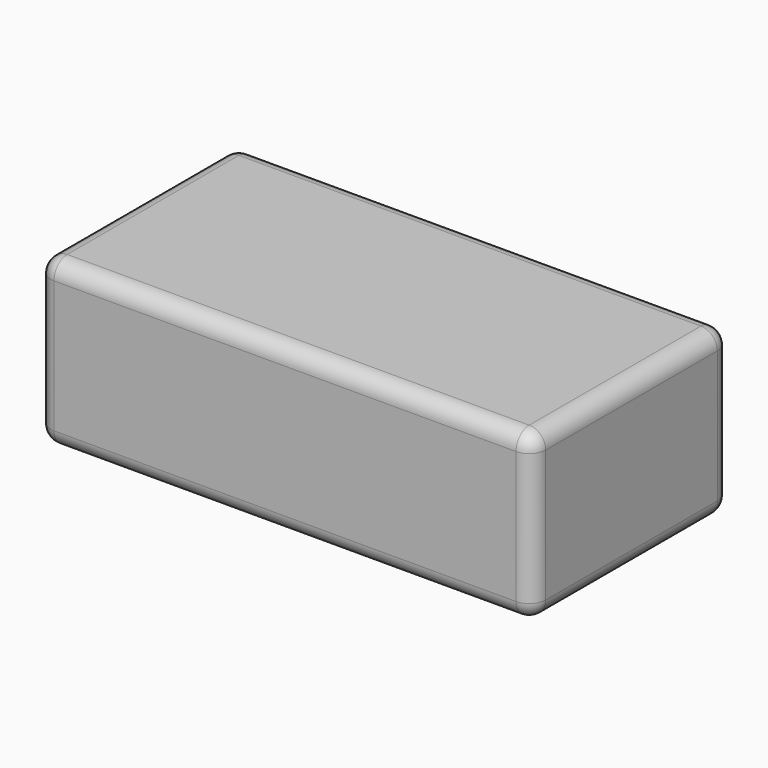
from build123d import *

# Parameters (mm, degrees)
F0_W          = 152.4
F0_H          = 76.2
F1_DEPTH      = 50.8
F2_R          = 18.0745305817
F3_DEPTH      = 38.1
F6_DEPTH      = 38.1
F4_W          = 35.56
F4_H          = 35.56
F7_DEPTH      = 38.1
F8_T1_DEPTH   = 35.56
F8_T3_DEPTH   = 35.56
F8_T5_DEPTH   = 142.24
F8_T7_DEPTH   = 66.04
F8_T9_DEPTH   = 40.64
F8_S13_W      = 5.08
F8_S13_H      = 5.08
F8_T14_DEPTH  = 5.08
F8_S19_W      = 5.08
F8_S19_H      = 5.08
F8_T20_DEPTH  = 5.08
F8_S25_W      = 5.08
F8_S25_H      = 5.08
F8_T26_DEPTH  = 5.08
F8_S31_W      = 5.08
F8_S31_H      = 5.08
F8_T32_DEPTH  = 5.08
F8_S37_W      = 5.08
F8_S37_H      = 5.08
F8_T38_DEPTH  = 5.08
F8_S43_W      = 5.08
F8_S43_H      = 5.08
F8_T44_DEPTH  = 5.08
F8_S49_W      = 5.08
F8_S49_H      = 5.08
F8_T50_DEPTH  = 5.08
F8_S55_W      = 5.08
F8_S55_H      = 5.08
F8_T56_DEPTH  = 5.08
F8_T64_DEPTH  = 64.7384888256
F8_T70_DEPTH  = 64.7384888256
F8_T76_DEPTH  = 55.6341915667
F8_T83_DEPTH  = 48.26
F8_T87_DEPTH  = 48.26
F8_T94_DEPTH  = 48.26
F8_T98_DEPTH  = 48.26
F8_T105_DEPTH = 48.26
F8_T109_DEPTH = 48.26
F8_T116_DEPTH = 48.26
F8_T120_DEPTH = 48.26
F8_T127_DEPTH = 64.7384888256
F8_T131_DEPTH = 55.6341915667
F8_T138_DEPTH = 64.7384888256
F8_T142_DEPTH = 64.7384888256
F8_T149_DEPTH = 55.6341915667
F8_T153_DEPTH = 64.7384888256


# Not quite as in the source:
# - a fillet or chamfer that OpenCascade refuses, or shapes differently, is made with other operations: its cross-section is extruded or revolved along the edge and cut away or added


with BuildPart() as f1:
    # F0 (on Top) → F1 (new body)
    with BuildSketch(Plane.XY):
        with Locations((1.4952687383, 0.1409448402)):
            Rectangle(F0_W, F0_H)
    extrude(amount=F1_DEPTH)

    # F2 (on Top) → F3 (cut)
    with BuildSketch(Plane.XY):
        with Locations((-49.4992733002, 0)):
            Circle(F2_R)
    extrude(amount=F3_DEPTH, mode=Mode.SUBTRACT)

    # F5 (on Top) → F6 (cut)
    with BuildSketch(Plane.XY):
        Polygon((50.7897567004, 18.7120139599), (35.672660917, 18.7120139599), (50.7897567004, -17.6058895886), align=None)
        Polygon((65.9068524837, 18.7120139599), (50.7897567004, 18.7120139599), (50.7897567004, -17.6058895886), align=None)
    extrude(amount=F6_DEPTH, mode=Mode.SUBTRACT)

    # F4 (on Top) → F7 (cut)
    with BuildSketch(Plane.XY):
        with Locations((1.4748377725, -0.014944126)):
            Rectangle(F4_W, F4_H)
    extrude(amount=F7_DEPTH, mode=Mode.SUBTRACT)

    # F8: fillet of radius 5.08 on 20 edges, made by hand

    # F8_s2 → F8_t1 (cut)
    with BuildSketch(Plane.YZ.offset(-16.3051622275)):
        with BuildLine():
            ThreePointArc((-22.874944126, 0), (-19.2828416775, 1.4878975516), (-17.794944126, 5.08))
            Line((-17.794944126, 5.08), (-17.794944126, 0))
            Line((-17.794944126, 0), (-22.874944126, 0))
        make_face()
        with BuildLine():
            ThreePointArc((22.845055874, 0), (19.2529534256, 1.4878975516), (17.765055874, 5.08))
            Line((17.765055874, 5.08), (17.765055874, 0))
            Line((17.765055874, 0), (22.845055874, 0))
        make_face()
    extrude(amount=F8_T1_DEPTH, mode=Mode.SUBTRACT)

    # F8_s4 → F8_t3 (cut)
    with BuildSketch(Plane.XZ.offset(-17.765055874)):
        with BuildLine():
            ThreePointArc((-21.3851622275, 0), (-17.793059779, 1.4878975516), (-16.3051622275, 5.08))
            Line((-16.3051622275, 5.08), (-16.3051622275, 0))
            Line((-16.3051622275, 0), (-21.3851622275, 0))
        make_face()
        with BuildLine():
            ThreePointArc((24.3348377725, 0), (20.7427353241, 1.4878975516), (19.2548377725, 5.08))
            Line((19.2548377725, 5.08), (19.2548377725, 0))
            Line((19.2548377725, 0), (24.3348377725, 0))
        make_face()
    extrude(amount=F8_T3_DEPTH, mode=Mode.SUBTRACT)

    # F8_s6 → F8_t5 (cut)
    with BuildSketch(Plane.YZ.offset(-69.6247312617)):
        with BuildLine():
            ThreePointArc((38.2409448402, 5.08), (36.7530472886, 1.4878975516), (33.1609448402, 0))
            Line((33.1609448402, 0), (38.2409448402, 0))
            Line((38.2409448402, 0), (38.2409448402, 5.08))
        make_face()
        with BuildLine():
            ThreePointArc((-32.8790551598, 0), (-36.4711576083, 1.4878975516), (-37.9590551598, 5.08))
            Line((-37.9590551598, 5.08), (-37.9590551598, 0))
            Line((-37.9590551598, 0), (-32.8790551598, 0))
        make_face()
        with BuildLine():
            ThreePointArc((38.2409448402, 45.72), (36.7530472886, 49.3121024484), (33.1609448402, 50.8))
            Line((33.1609448402, 50.8), (38.2409448402, 50.8))
            Line((38.2409448402, 50.8), (38.2409448402, 45.72))
        make_face()
        with BuildLine():
            ThreePointArc((-32.8790551598, 50.8), (-36.4711576083, 49.3121024484), (-37.9590551598, 45.72))
            Line((-37.9590551598, 45.72), (-37.9590551598, 50.8))
            Line((-37.9590551598, 50.8), (-32.8790551598, 50.8))
        make_face()
    extrude(amount=F8_T5_DEPTH, mode=Mode.SUBTRACT)

    # F8_s8 → F8_t7 (cut)
    with BuildSketch(Plane.XZ.offset(-33.1609448402)):
        with BuildLine():
            ThreePointArc((77.6952687383, 5.08), (76.2073711867, 1.4878975516), (72.6152687383, 0))
            Line((72.6152687383, 0), (77.6952687383, 0))
            Line((77.6952687383, 0), (77.6952687383, 5.08))
        make_face()
        with BuildLine():
            ThreePointArc((-74.7047312617, 5.08), (-73.2168337102, 1.4878975516), (-69.6247312617, 0))
            Line((-69.6247312617, 0), (-74.7047312617, 0))
            Line((-74.7047312617, 0), (-74.7047312617, 5.08))
        make_face()
        with BuildLine():
            ThreePointArc((-74.7047312617, 45.72), (-73.2168337102, 49.3121024484), (-69.6247312617, 50.8))
            Line((-69.6247312617, 50.8), (-74.7047312617, 50.8))
            Line((-74.7047312617, 50.8), (-74.7047312617, 45.72))
        make_face()
        with BuildLine():
            ThreePointArc((77.6952687383, 45.72), (76.2073711867, 49.3121024484), (72.6152687383, 50.8))
            Line((72.6152687383, 50.8), (77.6952687383, 50.8))
            Line((77.6952687383, 50.8), (77.6952687383, 45.72))
        make_face()
    extrude(amount=F8_T7_DEPTH, mode=Mode.SUBTRACT)

    # F8_s10 → F8_t9 (cut)
    with BuildSketch(Plane.XY.offset(5.08)):
        with BuildLine():
            ThreePointArc((72.6152687383, 38.2409448402), (76.2073711867, 36.7530472886), (77.6952687383, 33.1609448402))
            Line((77.6952687383, 33.1609448402), (77.6952687383, 38.2409448402))
            Line((77.6952687383, 38.2409448402), (72.6152687383, 38.2409448402))
        make_face()
        with BuildLine():
            ThreePointArc((77.6952687383, -32.8790551598), (76.2073711867, -36.4711576083), (72.6152687383, -37.9590551598))
            Line((72.6152687383, -37.9590551598), (77.6952687383, -37.9590551598))
            Line((77.6952687383, -37.9590551598), (77.6952687383, -32.8790551598))
        make_face()
        with BuildLine():
            ThreePointArc((-74.7047312617, -32.8790551598), (-73.2168337102, -36.4711576083), (-69.6247312617, -37.9590551598))
            Line((-69.6247312617, -37.9590551598), (-74.7047312617, -37.9590551598))
            Line((-74.7047312617, -37.9590551598), (-74.7047312617, -32.8790551598))
        make_face()
        with BuildLine():
            ThreePointArc((-69.6247312617, 38.2409448402), (-73.2168337102, 36.7530472886), (-74.7047312617, 33.1609448402))
            Line((-74.7047312617, 33.1609448402), (-74.7047312617, 38.2409448402))
            Line((-74.7047312617, 38.2409448402), (-69.6247312617, 38.2409448402))
        make_face()
    extrude(amount=F8_T9_DEPTH, mode=Mode.SUBTRACT)


with BuildPart() as f8_tool12:
    # F8_s13 → F8_t14 (new body)
    with BuildSketch(Plane.XZ.offset(-33.1609448402)):
        with Locations((75.1552687383, 2.54)):
            Rectangle(F8_S13_W, F8_S13_H)
    extrude(amount=-F8_T14_DEPTH)

    # F8_s15 → F8_t16 (revolve, cut)
    with BuildSketch(Plane(origin=(72.6152687383, 33.1609448402, 5.08), x_dir=(-0.7071067812, 0, 0.7071067812), z_dir=(-0.7071067812, 0, -0.7071067812))):
        with BuildLine():
            ThreePointArc((0, -5.08), (5.08, 0), (0, 5.08))
            Line((0, 5.08), (0, -5.08))
        make_face()
    revolve(axis=Axis((72.6152687383, 33.1609448402, 5.08), (0, 1, 0)), mode=Mode.SUBTRACT)


with BuildPart() as f1_1:
    add(f1.part)

    # F8_t11: cut F8_tool12
    add(f8_tool12.part, mode=Mode.SUBTRACT)


with BuildPart() as f8_tool18:
    # F8_s19 → F8_t20 (new body)
    with BuildSketch(Plane.XZ.offset(-33.1609448402)):
        with Locations((-72.1647312617, 2.54)):
            Rectangle(F8_S19_W, F8_S19_H)
    extrude(amount=-F8_T20_DEPTH)

    # F8_s21 → F8_t22 (revolve, cut)
    with BuildSketch(Plane(origin=(-69.6247312617, 33.1609448402, 5.08), x_dir=(0.7071067812, 0, 0.7071067812), z_dir=(-0.7071067812, 0, 0.7071067812))):
        with BuildLine():
            ThreePointArc((0, -5.08), (5.08, 0), (0, 5.08))
            Line((0, 5.08), (0, -5.08))
        make_face()
    revolve(axis=Axis((-69.6247312617, 33.1609448402, 5.08), (0, 1, 0)), mode=Mode.SUBTRACT)


with BuildPart() as f1_2:
    add(f1_1.part)

    # F8_t17: cut F8_tool18
    add(f8_tool18.part, mode=Mode.SUBTRACT)


with BuildPart() as f8_tool24:
    # F8_s25 → F8_t26 (new body)
    with BuildSketch(Plane.YZ.offset(72.6152687383)):
        with Locations((-35.4190551598, 2.54)):
            Rectangle(F8_S25_W, F8_S25_H)
    extrude(amount=F8_T26_DEPTH)

    # F8_s27 → F8_t28 (revolve, cut)
    with BuildSketch(Plane(origin=(72.6152687383, -32.8790551598, 5.08), x_dir=(0, 0.7071067812, 0.7071067812), z_dir=(0, 0.7071067812, -0.7071067812))):
        with BuildLine():
            ThreePointArc((0, -5.08), (5.08, 0), (0, 5.08))
            Line((0, 5.08), (0, -5.08))
        make_face()
    revolve(axis=Axis((72.6152687383, -32.8790551598, 5.08), (1, 0, 0)), mode=Mode.SUBTRACT)


with BuildPart() as f1_3:
    add(f1_2.part)

    # F8_t23: cut F8_tool24
    add(f8_tool24.part, mode=Mode.SUBTRACT)


with BuildPart() as f8_tool30:
    # F8_s31 → F8_t32 (new body)
    with BuildSketch(Plane.YZ.offset(-69.6247312617)):
        with Locations((-35.4190551598, 2.54)):
            Rectangle(F8_S31_W, F8_S31_H)
    extrude(amount=-F8_T32_DEPTH)

    # F8_s33 → F8_t34 (revolve, cut)
    with BuildSketch(Plane(origin=(-69.6247312617, -32.8790551598, 5.08), x_dir=(0, 0.7071067812, 0.7071067812), z_dir=(0, -0.7071067812, 0.7071067812))):
        with BuildLine():
            ThreePointArc((0, -5.08), (5.08, 0), (0, 5.08))
            Line((0, 5.08), (0, -5.08))
        make_face()
    revolve(axis=Axis((-69.6247312617, -32.8790551598, 5.08), (-1, 0, 0)), mode=Mode.SUBTRACT)


with BuildPart() as f1_4:
    add(f1_3.part)

    # F8_t29: cut F8_tool30
    add(f8_tool30.part, mode=Mode.SUBTRACT)


with BuildPart() as f8_tool36:
    # F8_s37 → F8_t38 (new body)
    with BuildSketch(Plane.XZ.offset(-33.1609448402)):
        with Locations((75.1552687383, 48.26)):
            Rectangle(F8_S37_W, F8_S37_H)
    extrude(amount=-F8_T38_DEPTH)

    # F8_s39 → F8_t40 (revolve, cut)
    with BuildSketch(Plane(origin=(72.6152687383, 33.1609448402, 45.72), x_dir=(-0.7071067812, 0, -0.7071067812), z_dir=(0.7071067812, 0, -0.7071067812))):
        with BuildLine():
            ThreePointArc((0, -5.08), (5.08, 0), (0, 5.08))
            Line((0, 5.08), (0, -5.08))
        make_face()
    revolve(axis=Axis((72.6152687383, 33.1609448402, 45.72), (0, 1, 0)), mode=Mode.SUBTRACT)


with BuildPart() as f1_5:
    add(f1_4.part)

    # F8_t35: cut F8_tool36
    add(f8_tool36.part, mode=Mode.SUBTRACT)


with BuildPart() as f8_tool42:
    # F8_s43 → F8_t44 (new body)
    with BuildSketch(Plane.YZ.offset(72.6152687383)):
        with Locations((-35.4190551598, 48.26)):
            Rectangle(F8_S43_W, F8_S43_H)
    extrude(amount=F8_T44_DEPTH)

    # F8_s45 → F8_t46 (revolve, cut)
    with BuildSketch(Plane(origin=(72.6152687383, -32.8790551598, 45.72), x_dir=(0, 0.7071067812, -0.7071067812), z_dir=(0, -0.7071067812, -0.7071067812))):
        with BuildLine():
            ThreePointArc((0, -5.08), (5.08, 0), (0, 5.08))
            Line((0, 5.08), (0, -5.08))
        make_face()
    revolve(axis=Axis((72.6152687383, -32.8790551598, 45.72), (1, 0, 0)), mode=Mode.SUBTRACT)


with BuildPart() as f1_6:
    add(f1_5.part)

    # F8_t41: cut F8_tool42
    add(f8_tool42.part, mode=Mode.SUBTRACT)


with BuildPart() as f8_tool48:
    # F8_s49 → F8_t50 (new body)
    with BuildSketch(Plane.YZ.offset(-69.6247312617)):
        with Locations((-35.4190551598, 48.26)):
            Rectangle(F8_S49_W, F8_S49_H)
    extrude(amount=-F8_T50_DEPTH)

    # F8_s51 → F8_t52 (revolve, cut)
    with BuildSketch(Plane(origin=(-69.6247312617, -32.8790551598, 45.72), x_dir=(0, 0.7071067812, -0.7071067812), z_dir=(0, 0.7071067812, 0.7071067812))):
        with BuildLine():
            ThreePointArc((0, -5.08), (5.08, 0), (0, 5.08))
            Line((0, 5.08), (0, -5.08))
        make_face()
    revolve(axis=Axis((-69.6247312617, -32.8790551598, 45.72), (-1, 0, 0)), mode=Mode.SUBTRACT)


with BuildPart() as f1_7:
    add(f1_6.part)

    # F8_t47: cut F8_tool48
    add(f8_tool48.part, mode=Mode.SUBTRACT)


with BuildPart() as f8_tool54:
    # F8_s55 → F8_t56 (new body)
    with BuildSketch(Plane.XZ.offset(-33.1609448402)):
        with Locations((-72.1647312617, 48.26)):
            Rectangle(F8_S55_W, F8_S55_H)
    extrude(amount=-F8_T56_DEPTH)

    # F8_s57 → F8_t58 (revolve, cut)
    with BuildSketch(Plane(origin=(-69.6247312617, 33.1609448402, 45.72), x_dir=(0.7071067812, 0, -0.7071067812), z_dir=(0.7071067812, 0, 0.7071067812))):
        with BuildLine():
            ThreePointArc((0, -5.08), (5.08, 0), (0, 5.08))
            Line((0, 5.08), (0, -5.08))
        make_face()
    revolve(axis=Axis((-69.6247312617, 33.1609448402, 45.72), (0, 1, 0)), mode=Mode.SUBTRACT)


with BuildPart() as f1_8:
    add(f1_7.part)

    # F8_t53: cut F8_tool54
    add(f8_tool54.part, mode=Mode.SUBTRACT)

    # F8_s59 → F8_t60 (revolve, cut)
    with BuildSketch(Plane.XZ):
        with BuildLine():
            ThreePointArc((-26.3447427184, 0), (-29.9368451669, 1.4878975516), (-31.4247427184, 5.08))
            Line((-31.4247427184, 5.08), (-31.4247427184, 0))
            Line((-31.4247427184, 0), (-26.3447427184, 0))
        make_face()
    revolve(axis=Axis((-49.4992733002, 0, 0), (0, 0, 1)), mode=Mode.SUBTRACT)


with BuildPart() as f8_tool62:
    # F8_s63 → F8_t64 (new body)
    with BuildSketch(Plane(origin=(-6.2510630726, 15.0177989873, 0), x_dir=(0, 0, 1), z_dir=(0.384282575, -0.9232155233, 0))):
        with BuildLine():
            ThreePointArc((0, -35.0442552258), (1.4878975516, -38.6363576742), (5.08, -40.1242552258))
            Line((5.08, -40.1242552258), (0, -40.1242552258))
            Line((0, -40.1242552258), (0, -35.0442552258))
        make_face()
    extrude(amount=F8_T64_DEPTH)

    split(bisect_by=Plane.XZ.offset(-18.7120139599), keep=Keep.TOP)

    split(bisect_by=Plane(origin=(49.535616731, -20.6188846174, 0), x_dir=(0, 0, 1), z_dir=(-0.9232155233, 0.384282575, 0)), keep=Keep.TOP)


with BuildPart() as f1_9:
    add(f1_8.part)

    # F8_t61: cut F8_tool62
    add(f8_tool62.part, mode=Mode.SUBTRACT)


with BuildPart() as f8_tool68:
    # F8_s69 → F8_t70 (new body)
    with BuildSketch(Plane(origin=(-3.6262487334, -8.7118421177, 0), x_dir=(0, 0, 1), z_dir=(0.384282575, 0.9232155233, 0))):
        with BuildLine():
            ThreePointArc((0, 58.7355283991), (1.4878975516, 55.1434259507), (5.08, 53.6555283991))
            Line((5.08, 53.6555283991), (0, 53.6555283991))
            Line((0, 53.6555283991), (0, 58.7355283991))
        make_face()
    extrude(amount=F8_T70_DEPTH)

    split(bisect_by=Plane(origin=(37.0433352869, 15.419052119, 0), x_dir=(0, 0, 1), z_dir=(0.9232155233, 0.384282575, 0)), keep=Keep.TOP)

    split(bisect_by=Plane.XZ.offset(-18.7120139599), keep=Keep.TOP)


with BuildPart() as f1_10:
    add(f1_9.part)

    # F8_t67: cut F8_tool68
    add(f8_tool68.part, mode=Mode.SUBTRACT)


with BuildPart() as f8_tool74:
    # F8_s75 → F8_t76 (new body)
    with BuildSketch(Plane.YZ.offset(78.6068524837)):
        with BuildLine():
            ThreePointArc((23.7920139599, 0), (20.1999115115, 1.4878975516), (18.7120139599, 5.08))
            Line((18.7120139599, 5.08), (18.7120139599, 0))
            Line((18.7120139599, 0), (23.7920139599, 0))
        make_face()
    extrude(amount=-F8_T76_DEPTH)

    split(bisect_by=Plane(origin=(37.0433352869, 15.419052119, 0), x_dir=(0, 0, 1), z_dir=(0.9232155233, 0.384282575, 0)), keep=Keep.TOP)

    split(bisect_by=Plane(origin=(49.535616731, -20.6188846174, 0), x_dir=(0, 0, 1), z_dir=(-0.9232155233, 0.384282575, 0)), keep=Keep.TOP)


with BuildPart() as f1_11:
    add(f1_10.part)

    # F8_t73: cut F8_tool74
    add(f8_tool74.part, mode=Mode.SUBTRACT)


with BuildPart() as f8_tool81:
    # F8_s82 → F8_t83 (new body)
    with BuildSketch(Plane.XZ.offset(-17.765055874)):
        with BuildLine():
            ThreePointArc((-21.3851622275, 0), (-17.793059779, 1.4878975516), (-16.3051622275, 5.08))
            Line((-16.3051622275, 5.08), (-16.3051622275, 0))
            Line((-16.3051622275, 0), (-21.3851622275, 0))
        make_face()
    extrude(amount=F8_T83_DEPTH)

    split(bisect_by=Plane.XZ.offset(17.794944126), keep=Keep.TOP)


with BuildPart() as f8_tool85:
    # F8_s86 → F8_t87 (new body)
    with BuildSketch(Plane.YZ.offset(-29.0051622275)):
        with BuildLine():
            ThreePointArc((-22.874944126, 0), (-19.2828416775, 1.4878975516), (-17.794944126, 5.08))
            Line((-17.794944126, 5.08), (-17.794944126, 0))
            Line((-17.794944126, 0), (-22.874944126, 0))
        make_face()
    extrude(amount=F8_T87_DEPTH)

    split(bisect_by=Plane.YZ.offset(-16.3051622275), keep=Keep.BOTTOM)


with BuildPart() as f8_tool81_1:
    add(f8_tool81.part)

    # F8_t89: intersect F8_tool85
    add(f8_tool85.part, mode=Mode.INTERSECT)


with BuildPart() as f1_12:
    add(f1_11.part)

    # F8_t79: cut F8_tool81
    add(f8_tool81_1.part, mode=Mode.SUBTRACT)


with BuildPart() as f8_tool92:
    # F8_s93 → F8_t94 (new body)
    with BuildSketch(Plane.YZ.offset(-16.3051622275)):
        with BuildLine():
            ThreePointArc((-22.874944126, 0), (-19.2828416775, 1.4878975516), (-17.794944126, 5.08))
            Line((-17.794944126, 5.08), (-17.794944126, 0))
            Line((-17.794944126, 0), (-22.874944126, 0))
        make_face()
    extrude(amount=F8_T94_DEPTH)

    split(bisect_by=Plane.YZ.offset(19.2548377725), keep=Keep.TOP)


with BuildPart() as f8_tool96:
    # F8_s97 → F8_t98 (new body)
    with BuildSketch(Plane.XZ.offset(30.494944126)):
        with BuildLine():
            ThreePointArc((24.3348377725, 0), (20.7427353241, 1.4878975516), (19.2548377725, 5.08))
            Line((19.2548377725, 5.08), (19.2548377725, 0))
            Line((19.2548377725, 0), (24.3348377725, 0))
        make_face()
    extrude(amount=-F8_T98_DEPTH)

    split(bisect_by=Plane.XZ.offset(17.794944126), keep=Keep.TOP)


with BuildPart() as f8_tool92_1:
    add(f8_tool92.part)

    # F8_t100: intersect F8_tool96
    add(f8_tool96.part, mode=Mode.INTERSECT)


with BuildPart() as f1_13:
    add(f1_12.part)

    # F8_t90: cut F8_tool92
    add(f8_tool92_1.part, mode=Mode.SUBTRACT)


with BuildPart() as f8_tool103:
    # F8_s104 → F8_t105 (new body)
    with BuildSketch(Plane.XZ.offset(-30.465055874)):
        with BuildLine():
            ThreePointArc((-21.3851622275, 0), (-17.793059779, 1.4878975516), (-16.3051622275, 5.08))
            Line((-16.3051622275, 5.08), (-16.3051622275, 0))
            Line((-16.3051622275, 0), (-21.3851622275, 0))
        make_face()
    extrude(amount=F8_T105_DEPTH)

    split(bisect_by=Plane.XZ.offset(-17.765055874), keep=Keep.BOTTOM)


with BuildPart() as f8_tool107:
    # F8_s108 → F8_t109 (new body)
    with BuildSketch(Plane.YZ.offset(19.2548377725)):
        with BuildLine():
            ThreePointArc((22.845055874, 0), (19.2529534256, 1.4878975516), (17.765055874, 5.08))
            Line((17.765055874, 5.08), (17.765055874, 0))
            Line((17.765055874, 0), (22.845055874, 0))
        make_face()
    extrude(amount=-F8_T109_DEPTH)

    split(bisect_by=Plane.YZ.offset(-16.3051622275), keep=Keep.BOTTOM)


with BuildPart() as f8_tool103_1:
    add(f8_tool103.part)

    # F8_t111: intersect F8_tool107
    add(f8_tool107.part, mode=Mode.INTERSECT)


with BuildPart() as f1_14:
    add(f1_13.part)

    # F8_t101: cut F8_tool103
    add(f8_tool103_1.part, mode=Mode.SUBTRACT)


with BuildPart() as f8_tool114:
    # F8_s115 → F8_t116 (new body)
    with BuildSketch(Plane.XZ.offset(17.794944126)):
        with BuildLine():
            ThreePointArc((24.3348377725, 0), (20.7427353241, 1.4878975516), (19.2548377725, 5.08))
            Line((19.2548377725, 5.08), (19.2548377725, 0))
            Line((19.2548377725, 0), (24.3348377725, 0))
        make_face()
    extrude(amount=-F8_T116_DEPTH)

    split(bisect_by=Plane.XZ.offset(-17.765055874), keep=Keep.BOTTOM)


with BuildPart() as f8_tool118:
    # F8_s119 → F8_t120 (new body)
    with BuildSketch(Plane.YZ.offset(31.9548377725)):
        with BuildLine():
            ThreePointArc((22.845055874, 0), (19.2529534256, 1.4878975516), (17.765055874, 5.08))
            Line((17.765055874, 5.08), (17.765055874, 0))
            Line((17.765055874, 0), (22.845055874, 0))
        make_face()
    extrude(amount=-F8_T120_DEPTH)

    split(bisect_by=Plane.YZ.offset(19.2548377725), keep=Keep.TOP)


with BuildPart() as f8_tool114_1:
    add(f8_tool114.part)

    # F8_t122: intersect F8_tool118
    add(f8_tool118.part, mode=Mode.INTERSECT)


with BuildPart() as f1_15:
    add(f1_14.part)

    # F8_t112: cut F8_tool114
    add(f8_tool114_1.part, mode=Mode.SUBTRACT)


with BuildPart() as f8_tool125:
    # F8_s126 → F8_t127 (new body)
    with BuildSketch(Plane(origin=(-6.2510630726, 15.0177989873, 0), x_dir=(0, 0, 1), z_dir=(0.384282575, -0.9232155233, 0))):
        with BuildLine():
            ThreePointArc((0, -35.0442552258), (1.4878975516, -38.6363576742), (5.08, -40.1242552258))
            Line((5.08, -40.1242552258), (0, -40.1242552258))
            Line((0, -40.1242552258), (0, -35.0442552258))
        make_face()
    extrude(amount=F8_T127_DEPTH)

    split(bisect_by=Plane.XZ.offset(-18.7120139599), keep=Keep.BOTTOM)


with BuildPart() as f8_tool129:
    # F8_s130 → F8_t131 (new body)
    with BuildSketch(Plane.YZ.offset(78.6068524837)):
        with BuildLine():
            ThreePointArc((23.7920139599, 0), (20.1999115115, 1.4878975516), (18.7120139599, 5.08))
            Line((18.7120139599, 5.08), (18.7120139599, 0))
            Line((18.7120139599, 0), (23.7920139599, 0))
        make_face()
    extrude(amount=-F8_T131_DEPTH)

    split(bisect_by=Plane(origin=(37.0433352869, 15.419052119, 0), x_dir=(0, 0, 1), z_dir=(-0.9232155233, -0.384282575, 0)), keep=Keep.TOP)


with BuildPart() as f8_tool125_1:
    add(f8_tool125.part)

    # F8_t133: intersect F8_tool129
    add(f8_tool129.part, mode=Mode.INTERSECT)


with BuildPart() as f1_16:
    add(f1_15.part)

    # F8_t123: cut F8_tool125
    add(f8_tool125_1.part, mode=Mode.SUBTRACT)


with BuildPart() as f8_tool136:
    # F8_s137 → F8_t138 (new body)
    with BuildSketch(Plane(origin=(-6.2510630726, 15.0177989873, 0), x_dir=(0, 0, 1), z_dir=(0.384282575, -0.9232155233, 0))):
        with BuildLine():
            ThreePointArc((0, -35.0442552258), (1.4878975516, -38.6363576742), (5.08, -40.1242552258))
            Line((5.08, -40.1242552258), (0, -40.1242552258))
            Line((0, -40.1242552258), (0, -35.0442552258))
        make_face()
    extrude(amount=F8_T138_DEPTH)

    split(bisect_by=Plane(origin=(49.535616731, -20.6188846174, 0), x_dir=(0, 0, 1), z_dir=(0.9232155233, -0.384282575, 0)), keep=Keep.TOP)


with BuildPart() as f8_tool140:
    # F8_s141 → F8_t142 (new body)
    with BuildSketch(Plane(origin=(-3.6262487334, -8.7118421177, 0), x_dir=(0, 0, 1), z_dir=(0.384282575, 0.9232155233, 0))):
        with BuildLine():
            ThreePointArc((0, 58.7355283991), (1.4878975516, 55.1434259507), (5.08, 53.6555283991))
            Line((5.08, 53.6555283991), (0, 53.6555283991))
            Line((0, 53.6555283991), (0, 58.7355283991))
        make_face()
    extrude(amount=F8_T142_DEPTH)

    split(bisect_by=Plane(origin=(37.0433352869, 15.419052119, 0), x_dir=(0, 0, 1), z_dir=(-0.9232155233, -0.384282575, 0)), keep=Keep.TOP)


with BuildPart() as f8_tool136_1:
    add(f8_tool136.part)

    # F8_t144: intersect F8_tool140
    add(f8_tool140.part, mode=Mode.INTERSECT)


with BuildPart() as f1_17:
    add(f1_16.part)

    # F8_t134: cut F8_tool136
    add(f8_tool136_1.part, mode=Mode.SUBTRACT)


with BuildPart() as f8_tool147:
    # F8_s148 → F8_t149 (new body)
    with BuildSketch(Plane.YZ.offset(78.6068524837)):
        with BuildLine():
            ThreePointArc((23.7920139599, 0), (20.1999115115, 1.4878975516), (18.7120139599, 5.08))
            Line((18.7120139599, 5.08), (18.7120139599, 0))
            Line((18.7120139599, 0), (23.7920139599, 0))
        make_face()
    extrude(amount=-F8_T149_DEPTH)

    split(bisect_by=Plane(origin=(49.535616731, -20.6188846174, 0), x_dir=(0, 0, 1), z_dir=(0.9232155233, -0.384282575, 0)), keep=Keep.TOP)


with BuildPart() as f8_tool151:
    # F8_s152 → F8_t153 (new body)
    with BuildSketch(Plane(origin=(-3.6262487334, -8.7118421177, 0), x_dir=(0, 0, 1), z_dir=(0.384282575, 0.9232155233, 0))):
        with BuildLine():
            ThreePointArc((0, 58.7355283991), (1.4878975516, 55.1434259507), (5.08, 53.6555283991))
            Line((5.08, 53.6555283991), (0, 53.6555283991))
            Line((0, 53.6555283991), (0, 58.7355283991))
        make_face()
    extrude(amount=F8_T153_DEPTH)

    split(bisect_by=Plane.XZ.offset(-18.7120139599), keep=Keep.BOTTOM)


with BuildPart() as f8_tool147_1:
    add(f8_tool147.part)

    # F8_t155: intersect F8_tool151
    add(f8_tool151.part, mode=Mode.INTERSECT)


with BuildPart() as f1_18:
    add(f1_17.part)

    # F8_t145: cut F8_tool147
    add(f8_tool147_1.part, mode=Mode.SUBTRACT)


solid = f1_18.part
